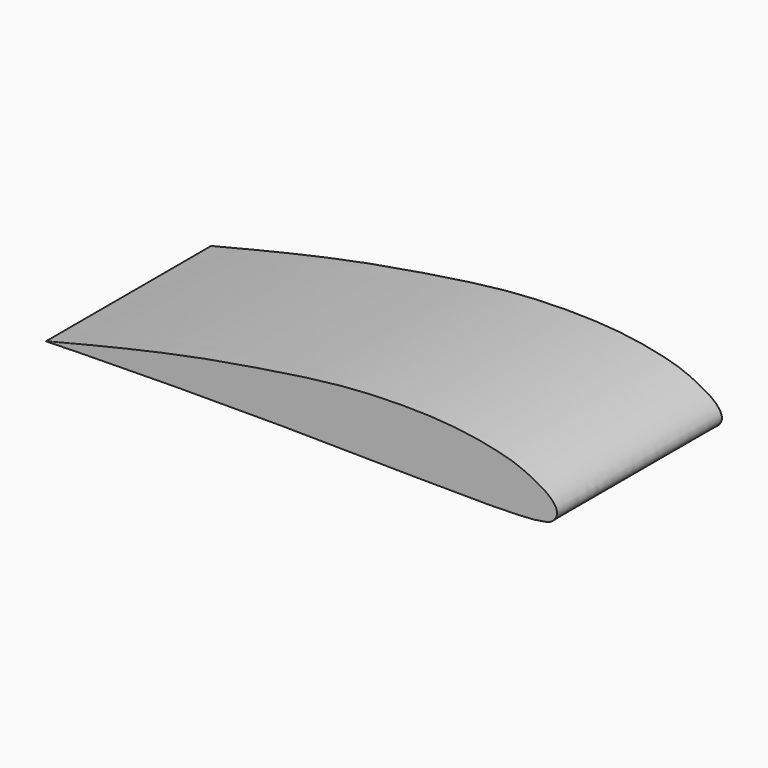
from build123d import *

# Parameters (mm, degrees)
F0_W     = 19.304
F0_H     = 6.604
F1_DEPTH = 76.2
F2_DEPTH = 6.604


# Not quite as in the source:
# - the dataset's text gives a spline's control points without its knots; the knots are read off the source's solid


with BuildPart() as f1:
    # F0 (on Front) → F1 (new body)
    with BuildSketch(Plane.XZ):
        with BuildLine():
            add(Edge.make_bspline(
                [(-116.1289155728, -8.8585806976), (-116.1004654569, -8.9214811682), (-113.3397440892, -8.8151818931), (-102.3185509608, -8.5511864998), (-58.9829552497, -7.8858156901), (-19.875847452, -8.1347627224), (-18.6797836816, -8.1476387653), (44.4665058995, -9.0989867527), (56.2339434046, -8.670038193), (63.7135209404, -8.4435378796), (68.4896594402, -7.6519341906), (69.719079739, -7.2821383509), (70.4809624753, -6.9336571594), (71.173343862, -6.4523170307), (71.776741831, -5.8576945919), (72.2069267863, -5.2715587783), (72.5013136464, -4.731477229), (72.6839882291, -4.2054709508), (72.7580639699, -3.8736193443), (72.805421114, -3.395728276), (72.7683512689, -2.9081998158), (72.6355276778, -2.3341468614), (72.383037615, -1.6774112328), (71.7953300256, -0.6970086124), (70.9643466539, 0.3018189632), (69.4405440762, 1.7041981277), (66.9875755216, 3.3424429063), (62.3302642741, 5.8392805943), (57.6853693281, 7.821371872), (52.5946429263, 9.2802515796), (45.0007549697, 10.9381118672), (36.7101489102, 12.189020725), (27.4758407757, 12.9679463985), (16.9450837638, 13.2238939186), (4.3554712464, 13.0078397844), (-7.8660448717, 12.0945082916), (-20.4511013859, 10.6035249255), (-40.400256883, 7.5442061765), (-60.7267686333, 4.0281167141), (-78.795557221, 0.1831405547), (-100.7921307643, -4.9306223816), (-113.2873605807, -8.2059737566), (-116.1578305779, -8.7946524014), (-116.1289155728, -8.8585806976)],
                knots=[0, 0, 0, 0, 0.0130491957, 0.0440066043, 0.1109645612, 0.1693650629, 0.1845200279, 0.2601585935, 0.297227308, 0.3222519534, 0.3432259075, 0.3538117117, 0.3623972714, 0.3712966115, 0.3802460949, 0.3885022479, 0.3961575709, 0.4032942665, 0.4089630871, 0.4155815182, 0.42240654, 0.4297507891, 0.4378777956, 0.4481278983, 0.459205589, 0.4728705156, 0.4895752088, 0.5119006412, 0.5337815859, 0.555985693, 0.5829463887, 0.6112137679, 0.6406139011, 0.6721764069, 0.7067075957, 0.7404524036, 0.7749091572, 0.8185379831, 0.8627452602, 0.9048194685, 0.9516457096, 0.9867375738, 1, 1, 1, 1], degree=3))
        make_face()
        with Locations((-50.7604071133, -2.1017281827)):
            Rectangle(F0_W, F0_H, mode=Mode.SUBTRACT)
        with Locations((52.4702374828, -1.5256585601)):
            Rectangle(F0_W, F0_H, mode=Mode.SUBTRACT)
        with Locations((1.6702374828, 3.8083414399)):
            Rectangle(F0_W, F0_H, mode=Mode.SUBTRACT)
        with Locations((-50.7604071133, -2.1017281827)):
            Rectangle(F0_W, F0_H)
        with Locations((1.6702374828, 3.8083414399)):
            Rectangle(F0_W, F0_H)
        with Locations((52.4702374828, -1.5256585601)):
            Rectangle(F0_W, F0_H)
    extrude(amount=F1_DEPTH)

    # F0 (on Front) → F2 (cut)
    with BuildSketch(Plane.XZ):
        with Locations((1.6702374828, 3.8083414399)):
            Rectangle(F0_W, F0_H)
        with Locations((52.4702374828, -1.5256585601)):
            Rectangle(F0_W, F0_H)
        with Locations((-50.7604071133, -2.1017281827)):
            Rectangle(F0_W, F0_H)
    extrude(amount=F2_DEPTH, mode=Mode.SUBTRACT)


solid = f1.part
